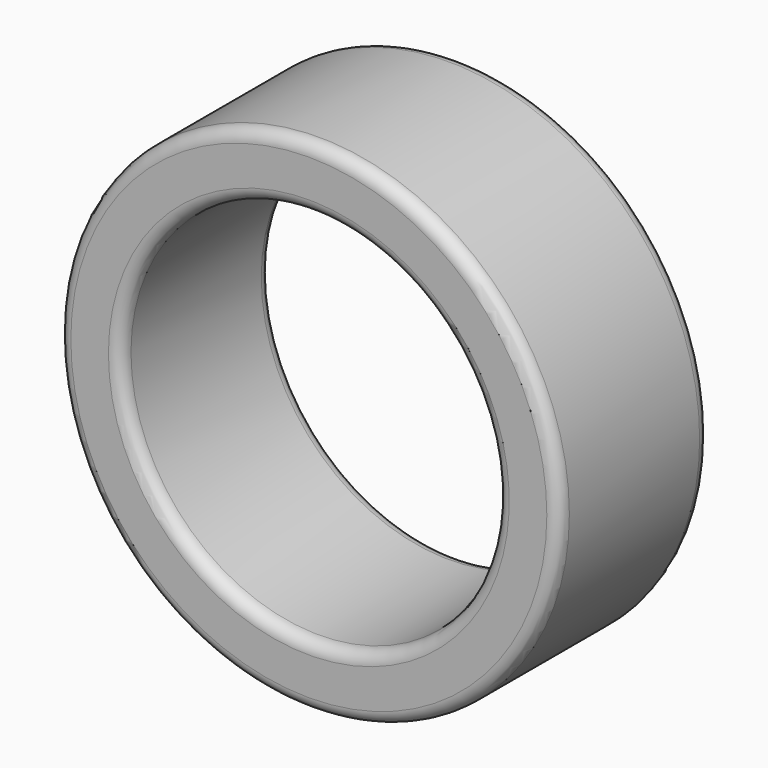
from build123d import *

# Parameters (mm, degrees)
F0_R     = 101.6
F1_DEPTH = 76.2
F3_D     = 152.4
F4_R     = 5.08


with BuildPart() as f1:
    # F0 (on Front) → F1 (new body)
    with BuildSketch(Plane.XZ):
        Circle(F0_R)
    extrude(amount=F1_DEPTH)

    # F3 (through all)
    with Locations(Plane.XZ.offset(76.2)):
        with Locations((0, 0)):
            Hole(F3_D / 2)

    # F4
    f4_edges = [f1.edges().sort_by_distance(p)[0] for p in [
        (-101.6, -76.2, 0),
        (-101.6, 0, 0),
        (-76.2, 0, 0),
        (-76.2, -76.2, 0),
    ]]
    fillet(f4_edges, radius=F4_R)


solid = f1.part
